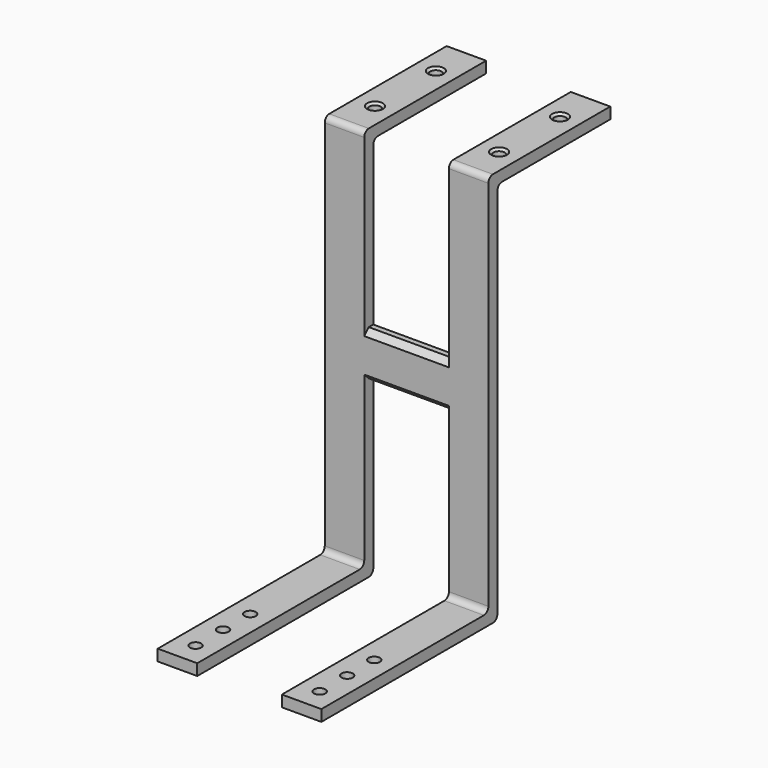
from build123d import *

# Parameters (mm, degrees)
F1_DEPTH = 10
F2_W     = 35
F2_H     = 10
F3_DEPTH = 185
F4_R     = 5
F5_DEPTH = 25
F6_W     = 35
F6_H     = 10
F7_DEPTH = 125
F8_R     = 5
F9_DEPTH = 25
F10_R    = 5
F11_SIZE = 5
F12_SIZE = 2


with BuildPart() as f1:
    # F0 (on Front) → F1 (new body)
    with BuildSketch(Plane.XZ):
        Polygon((-34.9524939805, 272.6582099839), (-69.9524939805, 272.6582099839), (-69.9524939805, -77.3417900161), (-34.9524939805, -77.3417900161), (-34.9524939805, 77.6582099839), (-34.9524939805, 97.6582099839), (-34.9524939805, 117.6582099839), align=None)
        Polygon((40.0475060195, 117.6582099839), (-34.9524939805, 117.6582099839), (-34.9524939805, 97.6582099839), (-34.9524939805, 77.6582099839), (40.0475060195, 77.6582099839), align=None)
        Polygon((40.0475060195, 272.6582099839), (40.0475060195, 117.6582099839), (40.0475060195, 77.6582099839), (40.0475060195, -77.3417900161), (75.0475060195, -77.3417900161), (75.0475060195, 272.6582099839), align=None)
    extrude(amount=F1_DEPTH)

    # F2 (on face) → F3 (join)
    with BuildSketch(Plane.XZ.offset(10)):
        with Locations((-52.4524939805, -72.3417900161)):
            Rectangle(F2_W, F2_H)
        with Locations((57.5475060195, -72.3417900161)):
            Rectangle(F2_W, F2_H)
    extrude(amount=F3_DEPTH)

    # F4 (on face) → F5 (cut)
    with BuildSketch(Plane.XY.offset(-67.3417900161)):
        with Locations((57.5475060195, -114.538833499)):
            Circle(F4_R)
        with Locations((57.5475060195, -144.5381194353)):
            Circle(F4_R)
        with Locations((57.5475060195, -175)):
            Circle(F4_R)
        with Locations((-52.4524939805, -114.538833499)):
            Circle(F4_R)
        with Locations((-52.4524939805, -144.5381194353)):
            Circle(F4_R)
        with Locations((-52.4524939805, -175)):
            Circle(F4_R)
    extrude(amount=-F5_DEPTH, mode=Mode.SUBTRACT)

    # F6 (on face) → F7 (join)
    with BuildSketch(Plane(origin=(0, 0, 0), x_dir=(-1, 0, 0), z_dir=(0, 1, 0))):
        with Locations((-57.5475060195, 267.6582099839)):
            Rectangle(F6_W, F6_H)
        with Locations((52.4524939805, 267.6582099839)):
            Rectangle(F6_W, F6_H)
    extrude(amount=F7_DEPTH)

    # F8 (on face) → F9 (cut)
    with BuildSketch(Plane.XY.offset(272.6582099839)):
        with Locations((-52.4524939805, 23.75)):
            Circle(F8_R)
        with Locations((-52.4524939805, 91.25)):
            Circle(F8_R)
        with Locations((57.5475060195, 91.25)):
            Circle(F8_R)
        with Locations((57.5475060195, 23.75)):
            Circle(F8_R)
    extrude(amount=-F9_DEPTH, mode=Mode.SUBTRACT)

    # F10
    f10_edges = [f1.edges().sort_by_distance(p)[0] for p in [
        (-52.452494, -10, 272.65821),
        (57.547506, -10, 272.65821),
        (-52.452494, -10, -67.34179),
        (57.547506, -10, -67.34179),
        (-52.452494, 0, -77.34179),
        (57.547506, 0, -77.34179),
        (-52.452494, 0, 262.65821),
        (57.547506, 0, 262.65821),
    ]]
    fillet(f10_edges, radius=F10_R)

    # F11
    f11_edges = [f1.edges().sort_by_distance(p)[0] for p in [
        (2.547506, -10, 77.65821),
        (2.547506, -10, 117.65821),
    ]]
    chamfer(f11_edges, length=F11_SIZE)

    # F12
    f12_edges = [f1.edges().sort_by_distance(p)[0] for p in [
        (52.547506, 23.75, 272.65821),
        (52.547506, 91.25, 272.65821),
        (-57.452494, 23.75, 272.65821),
        (-57.452494, 91.25, 272.65821),
        (-57.452494, -175, -77.34179),
        (-57.452494, -144.538119, -77.34179),
        (-57.452494, -114.538833, -77.34179),
        (52.547506, -114.538833, -77.34179),
        (52.547506, -144.538119, -77.34179),
        (52.547506, -175, -77.34179),
    ]]
    chamfer(f12_edges, length=F12_SIZE)


solid = f1.part
